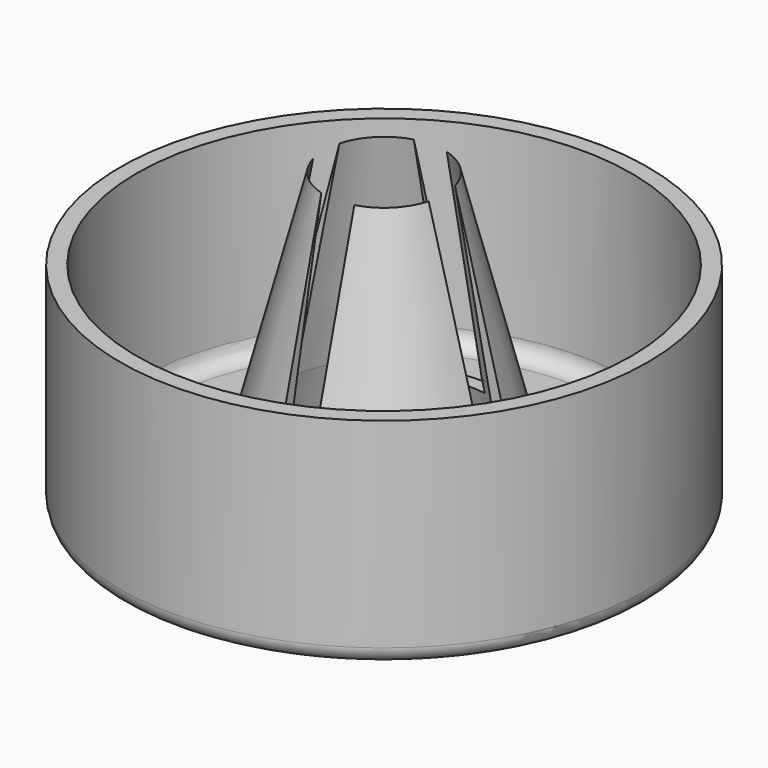
from build123d import *

# Parameters (mm, degrees)
F0_W         = 3.175
F0_H         = 38.1
F3_R         = 3.175
F4_W         = 3.175
F4_H         = 55.6163180947
F5_DEPTH     = 30.734
F6_W         = 3.175
F6_H         = 64.323036778
F7_DEPTH     = 27.178
F8_R         = 11.5282463958
F9_DEPTH     = 72.136
F10_T2_ANGLE = 359.64
F10_T4_ANGLE = 359.64
F10_T6_ANGLE = 359.64
F10_T8_ANGLE = 359.64


# Not quite as in the source:
# - a fillet or chamfer that OpenCascade refuses, or shapes differently, is made with other operations: its cross-section is extruded or revolved along the edge and cut away or added


with BuildPart() as f2:
    # F0 (on Front) → F2 (revolve)
    with BuildSketch(Plane.XZ):
        Polygon((7.1327639744, 64.2934367061), (23.8125, 0), (23.8125, 3.5723163746), (25.5098140885, 3.5723163746), (9.5913732515, 64.9312771426), align=None)
        Polygon((23.8125, 3.5723163746), (23.8125, 0), (50.8, 0), (50.8, 3.5723163746), (47.625, 3.5723163746), (25.5098140885, 3.5723163746), align=None)
        with Locations((49.2125, 22.6223163746)):
            Rectangle(F0_W, F0_H)
    revolve(axis=Axis((0, 0, 38.2007025182), (0, 0, 1)))

    # F3
    f3_edges = [f2.edges().sort_by_distance(p)[0] for p in [
        (-50.8, 0, 0),
        (-23.8125, 0, 0),
        (-25.509814, 0, 3.572316),
        (-47.625, 0, 3.572316),
    ]]
    fillet(f3_edges, radius=F3_R)

    # F4 (on Front) → F5 (cut, symmetric)
    with BuildSketch(Plane.XZ):
        with Locations((1.5875, 40.5081590474)):
            Rectangle(F4_W, F4_H)
        Polygon((-3.175, 12.7), (0, 12.7), (0, 68.3163180947), (0, 68.3765411377), (-3.175, 68.3765411377), align=None)
    extrude(amount=F5_DEPTH, both=True, mode=Mode.SUBTRACT)

    # F6 (on Right) → F7 (cut, symmetric)
    with BuildSketch(Plane.YZ):
        Polygon((0, 77.023036778), (0, 12.7), (3.175, 12.7), (3.175, 80.2117586136), (0, 80.2117586136), align=None)
        with Locations((-1.5875, 44.861518389)):
            Rectangle(F6_W, F6_H)
    extrude(amount=F7_DEPTH, both=True, mode=Mode.SUBTRACT)

    # F8 (on Top) → F9 (cut)
    with BuildSketch(Plane.XY):
        Circle(F8_R)
    extrude(amount=F9_DEPTH, mode=Mode.SUBTRACT)

    # F10: chamfer of 10.16 x 33.02 on 4 edges, made by hand

    # F10_s1 → F10_t2 (revolve, cut)
    with BuildSketch(Plane(origin=(0, 0, 0), x_dir=(0, 0, 1), z_dir=(-0.7093247296, -0.7048818539, 0))):
        Polygon((15.3887617085, 19.8201720703), (57.5106823112, 11.5282463958), (47.3506823112, 11.5282463958), align=None)
    revolve(axis=Axis((0, 0, 47.3506823112), (0, 0, -1)), revolution_arc=F10_T2_ANGLE, mode=Mode.SUBTRACT)

    # F10_s3 → F10_t4 (revolve, cut)
    with BuildSketch(Plane(origin=(0, 0, 0), x_dir=(0, 0, 1), z_dir=(-0.7048818539, 0.7093247296, 0))):
        Polygon((15.3887617085, 19.8201720703), (57.5106823112, 11.5282463958), (47.3506823112, 11.5282463958), align=None)
    revolve(axis=Axis((0, 0, 47.3506823112), (0, 0, -1)), revolution_arc=F10_T4_ANGLE, mode=Mode.SUBTRACT)

    # F10_s5 → F10_t6 (revolve, cut)
    with BuildSketch(Plane(origin=(0, 0, 0), x_dir=(0, 0, 1), z_dir=(0.7093247296, 0.7048818539, 0))):
        Polygon((15.3887617085, 19.8201720703), (57.5106823112, 11.5282463958), (47.3506823112, 11.5282463958), align=None)
    revolve(axis=Axis((0, 0, 47.3506823112), (0, 0, -1)), revolution_arc=F10_T6_ANGLE, mode=Mode.SUBTRACT)

    # F10_s7 → F10_t8 (revolve, cut)
    with BuildSketch(Plane(origin=(0, 0, 0), x_dir=(0, 0, 1), z_dir=(0.7048818539, -0.7093247296, 0))):
        Polygon((15.3887617085, 19.8201720703), (57.5106823112, 11.5282463958), (47.3506823112, 11.5282463958), align=None)
    revolve(axis=Axis((0, 0, 47.3506823112), (0, 0, -1)), revolution_arc=F10_T8_ANGLE, mode=Mode.SUBTRACT)


solid = f2.part
